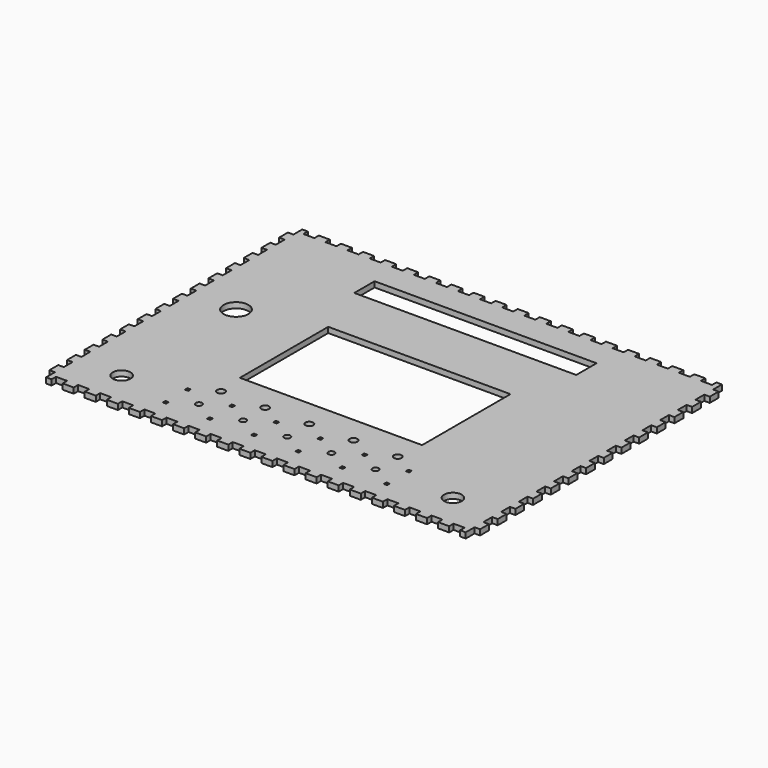
from build123d import *

# Parameters (mm, degrees)
F0_R     = 8
F0_W     = 3
F0_H     = 3
F0_R_2   = 2.85
F0_R_3   = 3.5
F0_W_2   = 165
F0_H_2   = 100
F0_R_4   = 11.25
F0_W_3   = 201
F0_H_3   = 23
F1_DEPTH = 2.5


# Not quite as in the source:
# - ends of sketch curves that miss each other by under 0.0002 mm in the source are joined


with BuildPart() as f1:
    # F0 (on Top) → F1 (new body, symmetric)
    with BuildSketch(Plane.XY):
        Polygon((-195, -125.0000041723), (-195, -135.0000041723), (-190, -135), (-190, -145), (-185, -145), (-185, -140), (-175, -140), (-175, -145), (-165, -145), (-165, -140), (-155, -140), (-155, -145), (-145, -145), (-145, -140), (-135, -140), (-135, -145), (-125, -145), (-125, -140), (-115, -140), (-115, -145), (-105, -145), (-105, -140), (-95, -140), (-95, -145), (-85, -145), (-85, -140), (-75, -140), (-75, -145), (-65, -145), (-65, -140), (-55, -140), (-55, -145), (-45, -145), (-45, -140), (-35, -140), (-35, -145), (-25, -145), (-25, -140), (-15, -140), (-15, -145), (-5, -145), (-5, -140), (5, -140), (5, -145), (15, -145), (15, -140), (25, -140), (25, -145), (35, -145), (35, -140), (45, -140), (45, -145), (55, -145), (55, -140), (65, -140), (65, -145), (75, -145), (75, -140), (85, -140), (85, -145), (95, -145), (95, -140), (105, -140), (105, -145), (115, -145), (115, -140), (125, -140), (125, -145), (135, -145), (135, -140), (145, -140), (145, -145), (155, -145), (155, -140), (165, -140), (165, -145), (175, -145), (175, -140), (185, -140), (185, -145), (190, -145), (190, -135), (195, -135), (194.9999928475, -125.0000041723), (189.9999928475, -125.0000041723), (189.9999928475, -115.0000041723), (194.9999928475, -115.0000041723), (194.9999928475, -105.0000041723), (189.9999928475, -105.0000041723), (189.9999928475, -95.0000041723), (194.9999928475, -95.0000041723), (194.9999928475, -85.0000041723), (189.9999928475, -85.0000041723), (189.9999928475, -75.0000041723), (194.9999928475, -75.0000041723), (194.9999928474, -65.0000041723), (189.9999928474, -65.0000041723), (189.9999928474, -55.0000041723), (195, -55.0000041723), (195, -45.0000041723), (190, -45.0000041723), (190, -35.0000041723), (194.9999928474, -35.0000041723), (194.9999928474, -25.0000041723), (189.9999928474, -25.0000041723), (189.9999928474, -15.0000041723), (194.9999928474, -15.0000041723), (194.9999928474, -5.0000041723), (189.9999928474, -5.0000041723), (189.9999928474, 4.9999958277), (194.9999928474, 4.9999958277), (194.9999928474, 14.9999958277), (189.9999928474, 14.9999958277), (189.9999928474, 24.9999958277), (194.9999928474, 24.9999958277), (194.9999928474, 34.9999958277), (189.9999928474, 34.9999958277), (189.9999928474, 44.9999958277), (194.9999928474, 44.9999958277), (194.9999928474, 54.9999958277), (189.9999928474, 54.9999958277), (189.9999928474, 64.9999958277), (194.9999928474, 64.9999958277), (194.9999928474, 74.9999958277), (189.9999928474, 74.9999958277), (189.9999928474, 84.9999958277), (194.9999928474, 84.9999958277), (194.9999928474, 94.9999958277), (189.9999928474, 94.9999958277), (189.9999928474, 104.9999958277), (194.9999928474, 104.9999958277), (194.9999928474, 114.9999958277), (189.9999928474, 114.9999958277), (189.9999928474, 124.9999958277), (194.9999928474, 124.9999958277), (194.9999928474, 134.9999958277), (190, 134.9999958277), (190, 144.9999958277), (185, 144.9999958277), (185, 139.9999958277), (175, 139.9999958277), (175, 144.9999958277), (165, 144.9999958277), (165, 139.9999958277), (155, 139.9999958277), (155, 144.9999958277), (145, 144.9999958277), (145, 139.9999958277), (135, 139.9999958277), (135, 144.9999958277), (125, 144.9999958277), (125, 139.9999958277), (115, 139.9999958277), (115, 144.9999958277), (105, 144.9999958277), (105, 139.9999958277), (95, 139.9999958277), (95, 144.9999958277), (85, 144.9999958277), (85, 139.9999958277), (75, 139.9999958277), (75, 144.9999958277), (65, 144.9999958277), (65, 139.9999958277), (55, 139.9999958277), (55, 144.9999958277), (45, 144.9999958277), (45, 139.9999958277), (35, 139.9999958277), (35, 144.9999958277), (25, 144.9999958277), (25, 139.9999958277), (15, 139.9999958277), (15, 144.9999958277), (5, 144.9999958277), (5, 139.9999958277), (-5, 139.9999958277), (-5, 144.9999958277), (-15, 144.9999958277), (-15, 139.9999958277), (-25, 139.9999958277), (-25, 144.9999958277), (-35, 144.9999958277), (-35, 139.9999958277), (-45, 139.9999958277), (-45, 144.9999958277), (-55, 144.9999958277), (-55, 139.9999958277), (-65, 139.9999958277), (-65, 144.9999958277), (-75, 144.9999958277), (-75, 139.9999958277), (-85, 139.9999958277), (-85, 144.9999958277), (-95, 144.9999958277), (-95, 139.9999958277), (-105, 139.9999958277), (-105, 144.9999958277), (-115, 144.9999958277), (-115, 139.9999958277), (-125, 139.9999958277), (-125, 144.9999958277), (-135, 144.9999958277), (-135, 139.9999958277), (-145, 139.9999958277), (-145, 144.9999958277), (-155, 144.9999958277), (-155, 139.9999958277), (-165, 139.9999958277), (-165, 144.9999958277), (-175, 144.9999958277), (-175, 139.9999958277), (-185, 139.9999958277), (-185, 144.9999958277), (-190, 144.9999958277), (-190, 134.9999958277), (-195, 134.9999958277), (-195, 124.9999958277), (-190, 124.9999958277), (-190, 114.9999958277), (-195, 114.9999958277), (-195, 104.9999958277), (-190, 104.9999958277), (-190, 94.9999958277), (-195, 94.9999958277), (-195, 84.9999958277), (-190, 84.9999958277), (-190, 74.9999958277), (-195, 74.9999958277), (-195, 64.9999958277), (-190, 64.9999958277), (-190, 54.9999958277), (-195, 54.9999958277), (-195, 44.9999958277), (-190, 44.9999958277), (-190, 34.9999958277), (-195, 34.9999958277), (-195, 24.9999958277), (-190, 24.9999958277), (-190, 14.9999958277), (-195, 14.9999958277), (-195, 4.9999958277), (-190, 4.9999958277), (-190, -5.0000041723), (-195, -5.0000041723), (-195, -15.0000041723), (-190, -15.0000041723), (-190, -25.0000041723), (-195, -25.0000041723), (-195, -35.0000041723), (-190, -35.0000041723), (-190, -45.0000041723), (-195, -45.0000041723), (-195, -55.0000041723), (-190, -55.0000041723), (-190, -65.0000041723), (-195, -65.0000041723), (-195, -75.0000041723), (-190, -75.0000041723), (-190, -85.0000041723), (-195, -85.0000041723), (-195, -95.0000041723), (-190, -95.0000041723), (-190, -105.0000041723), (-195, -105.0000041723), (-195, -115.0000041723), (-190, -115.0000041723), (-190, -125.0000041723), align=None)
        with Locations((-150, -109.5)):
            Circle(F0_R, mode=Mode.SUBTRACT)
        with Locations((-100, -122)):
            Rectangle(F0_W, F0_H, mode=Mode.SUBTRACT)
        with Locations((-100, -97)):
            Rectangle(F0_W, F0_H, mode=Mode.SUBTRACT)
        with Locations((-80, -109.5)):
            Circle(F0_R_2, mode=Mode.SUBTRACT)
        with Locations((-60, -122)):
            Rectangle(F0_W, F0_H, mode=Mode.SUBTRACT)
        with Locations((-40, -109.5)):
            Circle(F0_R_2, mode=Mode.SUBTRACT)
        with Locations((-20, -122)):
            Rectangle(F0_W, F0_H, mode=Mode.SUBTRACT)
        with Locations((-60, -97)):
            Rectangle(F0_W, F0_H, mode=Mode.SUBTRACT)
        with Locations((-80, -84.5)):
            Circle(F0_R_3, mode=Mode.SUBTRACT)
        with Locations((-20, -97)):
            Rectangle(F0_W, F0_H, mode=Mode.SUBTRACT)
        with Locations((-40, -84.5)):
            Circle(F0_R_3, mode=Mode.SUBTRACT)
        with Locations((20, -122)):
            Rectangle(F0_W, F0_H, mode=Mode.SUBTRACT)
        with Locations((0, -109.5)):
            Circle(F0_R_2, mode=Mode.SUBTRACT)
        with Locations((40, -109.5)):
            Circle(F0_R_2, mode=Mode.SUBTRACT)
        with Locations((60, -122)):
            Rectangle(F0_W, F0_H, mode=Mode.SUBTRACT)
        with Locations((80, -109.5)):
            Circle(F0_R_2, mode=Mode.SUBTRACT)
        with Locations((20, -97)):
            Rectangle(F0_W, F0_H, mode=Mode.SUBTRACT)
        with Locations((0, -84.5)):
            Circle(F0_R_3, mode=Mode.SUBTRACT)
        with Locations((40, -84.5)):
            Circle(F0_R_3, mode=Mode.SUBTRACT)
        with Locations((60, -97)):
            Rectangle(F0_W, F0_H, mode=Mode.SUBTRACT)
        with Locations((80, -84.5)):
            Circle(F0_R_3, mode=Mode.SUBTRACT)
        with Locations((100, -121.8875438174)):
            Rectangle(F0_W, F0_H, mode=Mode.SUBTRACT)
        with Locations((150, -109.5)):
            Circle(F0_R, mode=Mode.SUBTRACT)
        with Locations((100, -96.8875438174)):
            Rectangle(F0_W, F0_H, mode=Mode.SUBTRACT)
        with Locations((0, -10)):
            Rectangle(F0_W_2, F0_H_2, mode=Mode.SUBTRACT)
        with Locations((-150, 20)):
            Circle(F0_R_4, mode=Mode.SUBTRACT)
        with Locations((0, 103.5)):
            Rectangle(F0_W_3, F0_H_3, mode=Mode.SUBTRACT)
    extrude(amount=F1_DEPTH, both=True)


solid = f1.part
